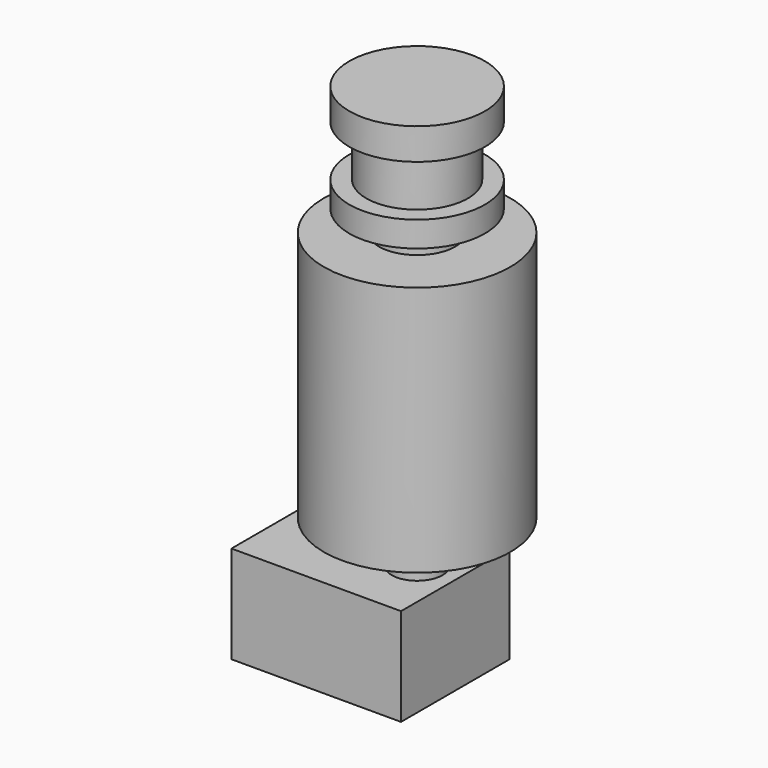
from build123d import *

# Parameters (mm, degrees)
F2_W     = 20
F2_H     = 16
F3_DEPTH = 11.5
F4_R     = 3


# Not quite as in the source:
# - an extrude whose draft closes it to a point is written as a loft to that point


with BuildPart() as f1:
    # F0 (on Front) → F1 (revolve)
    with BuildSketch(Plane.XZ):
        Polygon((0, -49.8), (0, 0), (-8, 0), (-8, -3.7), (-6, -3.7), (-6, -9.7), (-8, -9.7), (-8, -12.7), (-4.5, -12.7), (-4.5, -15.2), (-11, -15.2), (-11, -44.8), (-3, -44.8), (-3, -49.8), align=None)
    revolve(axis=Axis((0, 0, -24.9), (0, 0, -1)))

    # F2 (on face) → F3 (join)
    with BuildSketch(Plane(origin=(0, 0, -49.8), x_dir=(1, 0, 0), z_dir=(0, 0, -1))):
        with Locations((-5.5, 0)):
            Rectangle(F2_W, F2_H)
    extrude(amount=F3_DEPTH)

    # F4 (on face) → F5 section 0
    with BuildSketch(Plane(origin=(0, 0, -61.3), x_dir=(1, 0, 0), z_dir=(0, 0, -1)), mode=Mode.PRIVATE) as f5_s0:
        Circle(F4_R)
    loft([f5_s0.sketch, Vertex(0, 0, -64.3)], ruled=True)


solid = f1.part
